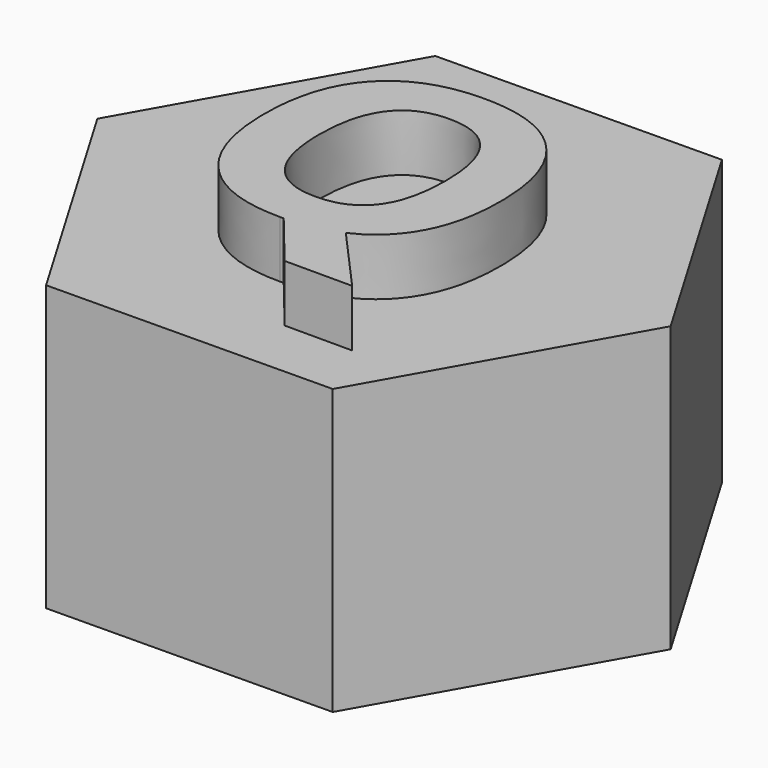
from build123d import *

# Parameters (mm, degrees)
F1_DEPTH     = 12.7
F2_TEXT_SIZE = 15.5519209661
F3_DEPTH     = 2.54


# Not quite as in the source:
# - Text() gives the source's letters only with a copy of the font that has no kerning and outlines rounded to 1/6400 em; it was checked with that copy


with BuildPart() as f1:
    # F0 (on Top) → F1 (new body)
    with BuildSketch(Plane.XY):
        Polygon((12.6993846473, 0.1250183213), (6.2414232815, 11.0604988776), (-6.4579613658, 10.9354805563), (-12.6993846473, -0.1250183213), (-6.2414232815, -11.0604988776), (6.4579613658, -10.9354805563), align=None)
    extrude(amount=F1_DEPTH)

    # F2 (on face) → F3 (join)
    with BuildSketch(Plane.XY.offset(12.7)):
        with Locations((-6.2414232815, -5.5986915478)):
            Text('Q', F2_TEXT_SIZE, font='Open Sans', font_style=FontStyle.BOLD, text_align=(TextAlign.LEFT, TextAlign.BOTTOM))
    extrude(amount=F3_DEPTH)


solid = f1.part
